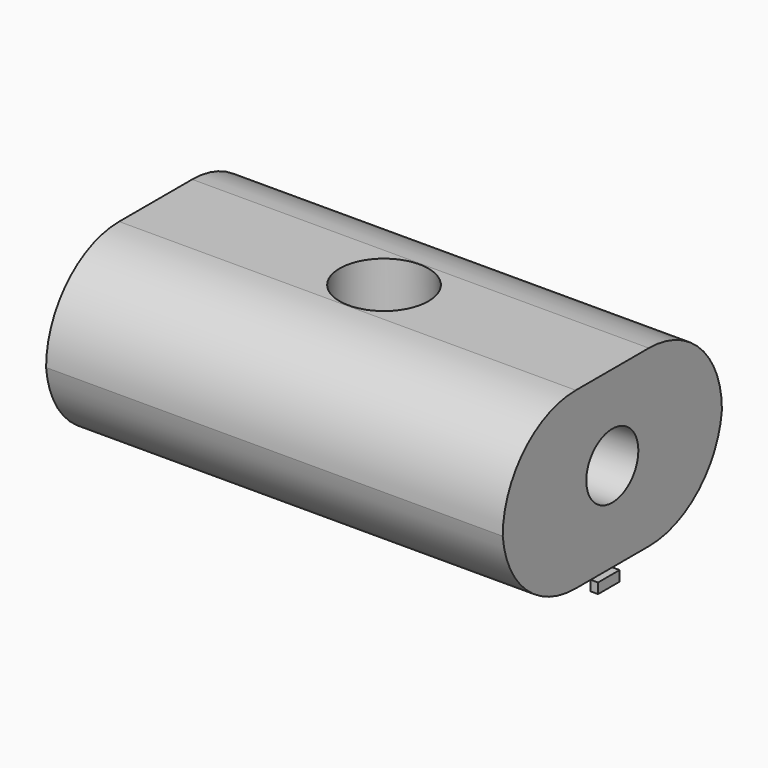
from build123d import *

# Parameters (mm, degrees)
F0_W        = 127
F0_H        = 76.2
F1_DEPTH    = 48.514
F2_R        = 25.4
F3_T1_DEPTH = 253.4846042015
F3_T3_DEPTH = 254
F4_T1_DEPTH = 253.4846042015
F5_W        = 7.5038918294
F5_H        = 2.8549211565
F6_DEPTH    = 2.032
F7_W        = 9.6475789323
F7_H        = 18.1432091631
F8_DEPTH    = 16
F9_W        = 5.6157563813
F9_H        = 8.6396243423
F10_DEPTH   = 16
F11_R       = 9.0424254563
F12_DEPTH   = 16
F13_R       = 12.7632843375
F14_DEPTH   = 16
F15_R       = 12.3503086405
F16_DEPTH   = 16
F17_R       = 4.9563337245
F18_DEPTH   = 1


# Not quite as in the source:
# - a fillet or chamfer that OpenCascade refuses, or shapes differently, is made with other operations: its cross-section is extruded or revolved along the edge and cut away or added


with BuildPart() as f1:
    # F0 (on Top) → F1 (new body)
    with BuildSketch(Plane.XY):
        Rectangle(F0_W, F0_H)
    extrude(amount=F1_DEPTH)

    # F2
    f2_edges = [f1.edges().sort_by_distance(p)[0] for p in [
        (0, -38.1, 48.514),
    ]]
    fillet(f2_edges, radius=F2_R)

    # F3: fillet of radius 25.4 on 2 edges, made by hand

    # F3_s2 → F3_t1 (cut)
    with BuildSketch(Plane.YZ.offset(-126.7423021007)):
        with BuildLine():
            ThreePointArc((-38.1, 23.114), (-29.936315865, 6.6486747135), (-12.8030791597, 0))
            Line((-12.8030791597, 0), (-38.1, 0))
            Line((-38.1, 0), (-38.1, 23.114))
        make_face()
    extrude(amount=F3_T1_DEPTH, mode=Mode.SUBTRACT)

    # F3_s4 → F3_t3 (cut)
    with BuildSketch(Plane.YZ.offset(-127)):
        with BuildLine():
            ThreePointArc((12.7, 48.514), (30.6605122421, 41.0745122421), (38.1, 23.114))
            Line((38.1, 23.114), (38.1, 48.514))
            Line((38.1, 48.514), (12.7, 48.514))
        make_face()
    extrude(amount=F3_T3_DEPTH, mode=Mode.SUBTRACT)

    # F4: fillet of radius 25.4 on 1 edges, made by hand

    # F4_s2 → F4_t1 (cut)
    with BuildSketch(Plane.YZ.offset(-126.7423021007)):
        with BuildLine():
            ThreePointArc((38.1, 23.114), (29.936315865, 6.6486747135), (12.8030791597, 0))
            Line((12.8030791597, 0), (38.1, 0))
            Line((38.1, 0), (38.1, 23.114))
        make_face()
    extrude(amount=F4_T1_DEPTH, mode=Mode.SUBTRACT)

    # F5 (on face) + F1_face1 (on face) → F6 (join)
    with BuildSketch(Plane.YZ.offset(63.5)):
        with Locations((-3.7519459147, -1.4274605783)):
            Rectangle(F5_W, F5_H)
    with BuildSketch(Plane(origin=(-63.5, 0, 24.2377466976), x_dir=(0, -1, 0), z_dir=(-1, 0, 0))):
        with BuildLine():
            ThreePointArc((38.1, -1.1237466976), (30.6605122421, 16.8367655446), (12.7, 24.2762533024))
            Line((12.7, 24.2762533024), (-12.7, 24.2762533024))
            ThreePointArc((-12.7, 24.2762533024), (-30.6605122421, 16.8367655445), (-38.1, -1.1237466976))
            ThreePointArc((-38.1, -1.1237466976), (-29.936315865, -17.5890719841), (-12.8030791597, -24.2377466976))
            Line((-12.8030791597, -24.2377466976), (12.8030791597, -24.2377466976))
            ThreePointArc((12.8030791597, -24.2377466976), (29.936315865, -17.5890719841), (38.1, -1.1237466976))
        make_face()
    extrude(amount=F6_DEPTH, dir=(1, 0, 0))

    # F7 (on face) → F8 (cut)
    with BuildSketch(Plane(origin=(-63.5, 0, 0), x_dir=(0, -1, 0), z_dir=(-1, 0, 0))):
        with Locations((-4.8237894662, 15.7912082504)):
            Rectangle(F7_W, F7_H)
    extrude(amount=-F8_DEPTH, mode=Mode.SUBTRACT)

    # F9 (on face) → F10 (cut)
    with BuildSketch(Plane(origin=(-63.5, 0, 0), x_dir=(0, -1, 0), z_dir=(-1, 0, 0))):
        with Locations((-2.8078781907, 32.6384725049)):
            Rectangle(F9_W, F9_H)
    extrude(amount=-F10_DEPTH, mode=Mode.SUBTRACT)

    # F11 (on face) → F12 (cut)
    with BuildSketch(Plane.YZ.offset(63.5)):
        with Locations((0, 24.896575138)):
            Circle(F11_R)
    extrude(amount=-F12_DEPTH, mode=Mode.SUBTRACT)

    # F13 (on face) → F14 (cut)
    with BuildSketch(Plane(origin=(0, 0, 0), x_dir=(1, 0, 0), z_dir=(0, 0, -1))):
        Circle(F13_R)
    extrude(amount=-F14_DEPTH, mode=Mode.SUBTRACT)

    # F15 (on face) → F16 (cut)
    with BuildSketch(Plane.XY.offset(48.514)):
        Circle(F15_R)
    extrude(amount=-F16_DEPTH, mode=Mode.SUBTRACT)

    # F17 (on face) → F18 (join)
    with BuildSketch(Plane.XY.offset(48.514)):
        with Locations((-48.0436608195, 0)):
            Circle(F17_R)
    extrude(amount=-F18_DEPTH)


solid = f1.part
